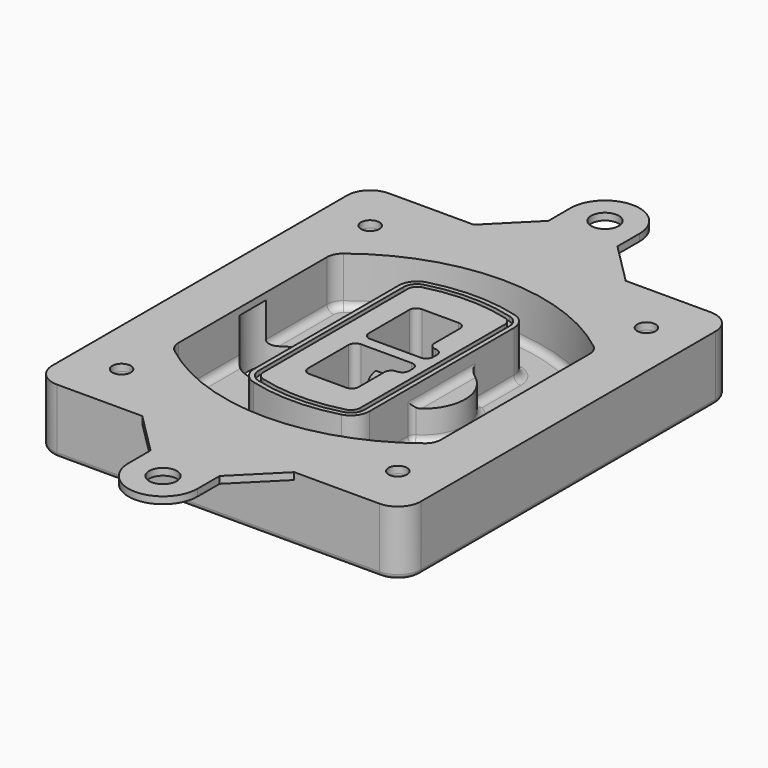
from build123d import *

# Parameters (mm, degrees)
F0_R      = 4
F1_DEPTH  = 25
F2_DEPTH  = 3
F3_DEPTH  = 18
F5_DEPTH  = 21
F6_DEPTH  = 2
F8_DEPTH  = 20
F9_DEPTH  = 16
F10_DEPTH = 25
F7_R      = 6
F7_R_2    = 4
F11_DEPTH = 6
F13_DEPTH = 9
F14_R     = 3
F15_R     = 2
F16_R     = 6
F16_R_2   = 4
F17_DEPTH = 3


with BuildPart() as f1:
    # F0 (on Top) → F1 (new body)
    with BuildSketch(Plane.XY):
        with BuildLine():
            ThreePointArc((-80, -80), (-77.0710678119, -87.0710678119), (-70, -90))
            Line((-70, -90), (70, -90))
            ThreePointArc((70, -90), (77.0710678119, -87.0710678119), (80, -80))
            Line((80, -80), (80, 80))
            ThreePointArc((80, 80), (77.0710678119, 87.0710678119), (70, 90))
            Line((70, 90), (-70, 90))
            ThreePointArc((-70, 90), (-77.0710678119, 87.0710678119), (-80, 80))
            Line((-80, 80), (-80, -80))
        make_face()
        with Locations((-60, -67.5)):
            Circle(F0_R, mode=Mode.SUBTRACT)
        with Locations((60, -67.5)):
            Circle(F0_R, mode=Mode.SUBTRACT)
        with Locations((-60, 67.5)):
            Circle(F0_R, mode=Mode.SUBTRACT)
        with BuildLine():
            ThreePointArc((-64, 40.2934422872), (-62.5820384798, 46.4328484224), (-58.6153846154, 51.3286200352))
            ThreePointArc((-58.6153846154, 51.3286200352), (0, 71.5), (58.6153846154, 51.3286200352))
            ThreePointArc((58.6153846154, 51.3286200352), (62.5820384798, 46.4328484224), (64, 40.2934422872))
            Line((64, 40.2934422872), (64, -40.2934422872))
            ThreePointArc((64, -40.2934422872), (62.5820384798, -46.4328484224), (58.6153846154, -51.3286200352))
            ThreePointArc((58.6153846154, -51.3286200352), (0, -71.5), (-58.6153846154, -51.3286200352))
            ThreePointArc((-58.6153846154, -51.3286200352), (-62.5820384798, -46.4328484224), (-64, -40.2934422872))
            Line((-64, -40.2934422872), (-64, 40.2934422872))
        make_face(mode=Mode.SUBTRACT)
        with Locations((60, 67.5)):
            Circle(F0_R, mode=Mode.SUBTRACT)
        with BuildLine():
            ThreePointArc((58.6153846154, 51.3286200352), (0, 71.5), (-58.6153846154, 51.3286200352))
            ThreePointArc((-58.6153846154, 51.3286200352), (-62.5820384798, 46.4328484224), (-64, 40.2934422872))
            Line((-64, 40.2934422872), (-64, -40.2934422872))
            ThreePointArc((-64, -40.2934422872), (-62.5820384798, -46.4328484224), (-58.6153846154, -51.3286200352))
            ThreePointArc((-58.6153846154, -51.3286200352), (0, -71.5), (58.6153846154, -51.3286200352))
            ThreePointArc((58.6153846154, -51.3286200352), (62.5820384798, -46.4328484224), (64, -40.2934422872))
            Line((64, -40.2934422872), (64, 40.2934422872))
            ThreePointArc((64, 40.2934422872), (62.5820384798, 46.4328484224), (58.6153846154, 51.3286200352))
        make_face()
        with BuildLine():
            Line((-60, -40.2934422872), (-60, 40.2934422872))
            ThreePointArc((-60, 40.2934422872), (-58.9871703427, 44.6787323838), (-56.1538461538, 48.1757121072))
            ThreePointArc((-56.1538461538, 48.1757121072), (0, 67.5), (56.1538461538, 48.1757121072))
            ThreePointArc((56.1538461538, 48.1757121072), (58.9871703427, 44.6787323838), (60, 40.2934422872))
            Line((60, 40.2934422872), (60, -40.2934422872))
            ThreePointArc((60, -40.2934422872), (58.9871703427, -44.6787323838), (56.1538461538, -48.1757121072))
            ThreePointArc((56.1538461538, -48.1757121072), (0, -67.5), (-56.1538461538, -48.1757121072))
            ThreePointArc((-56.1538461538, -48.1757121072), (-58.9871703427, -44.6787323838), (-60, -40.2934422872))
        make_face(mode=Mode.SUBTRACT)
        with BuildLine():
            ThreePointArc((-56.1538461538, 48.1757121072), (-58.9871703427, 44.6787323838), (-60, 40.2934422872))
            Line((-60, 40.2934422872), (-60, -40.2934422872))
            ThreePointArc((-60, -40.2934422872), (-58.9871703427, -44.6787323838), (-56.1538461538, -48.1757121072))
            ThreePointArc((-56.1538461538, -48.1757121072), (0, -67.5), (56.1538461538, -48.1757121072))
            ThreePointArc((56.1538461538, -48.1757121072), (58.9871703427, -44.6787323838), (60, -40.2934422872))
            Line((60, -40.2934422872), (60, 40.2934422872))
            ThreePointArc((60, 40.2934422872), (58.9871703427, 44.6787323838), (56.1538461538, 48.1757121072))
            ThreePointArc((56.1538461538, 48.1757121072), (0, 67.5), (-56.1538461538, 48.1757121072))
        make_face()
        with BuildLine():
            ThreePointArc((54.3076923077, 45.8110311612), (56.2910192399, 43.3631453548), (57, 40.2934422872))
            Line((57, 40.2934422872), (57, -40.2934422872))
            ThreePointArc((57, -40.2934422872), (56.2910192399, -43.3631453548), (54.3076923077, -45.8110311612))
            ThreePointArc((54.3076923077, -45.8110311612), (0, -64.5), (-54.3076923077, -45.8110311612))
            ThreePointArc((-54.3076923077, -45.8110311612), (-56.2910192399, -43.3631453548), (-57, -40.2934422872))
            Line((-57, -40.2934422872), (-57, 40.2934422872))
            ThreePointArc((-57, 40.2934422872), (-56.2910192399, 43.3631453548), (-54.3076923077, 45.8110311612))
            ThreePointArc((-54.3076923077, 45.8110311612), (0, 64.5), (54.3076923077, 45.8110311612))
        make_face(mode=Mode.SUBTRACT)
        with BuildLine():
            Line((57, -40.2934422872), (57, 40.2934422872))
            ThreePointArc((57, 40.2934422872), (56.2910192399, 43.3631453548), (54.3076923077, 45.8110311612))
            ThreePointArc((54.3076923077, 45.8110311612), (0, 64.5), (-54.3076923077, 45.8110311612))
            ThreePointArc((-54.3076923077, 45.8110311612), (-56.2910192399, 43.3631453548), (-57, 40.2934422872))
            Line((-57, 40.2934422872), (-57, -40.2934422872))
            ThreePointArc((-57, -40.2934422872), (-56.2910192399, -43.3631453548), (-54.3076923077, -45.8110311612))
            ThreePointArc((-54.3076923077, -45.8110311612), (0, -64.5), (54.3076923077, -45.8110311612))
            ThreePointArc((54.3076923077, -45.8110311612), (56.2910192399, -43.3631453548), (57, -40.2934422872))
        make_face()
    extrude(amount=-F1_DEPTH)

    # F0 (on Top) → F2 (join)
    with BuildSketch(Plane.XY):
        with BuildLine():
            ThreePointArc((-56.1538461538, 48.1757121072), (-58.9871703427, 44.6787323838), (-60, 40.2934422872))
            Line((-60, 40.2934422872), (-60, -40.2934422872))
            ThreePointArc((-60, -40.2934422872), (-58.9871703427, -44.6787323838), (-56.1538461538, -48.1757121072))
            ThreePointArc((-56.1538461538, -48.1757121072), (0, -67.5), (56.1538461538, -48.1757121072))
            ThreePointArc((56.1538461538, -48.1757121072), (58.9871703427, -44.6787323838), (60, -40.2934422872))
            Line((60, -40.2934422872), (60, 40.2934422872))
            ThreePointArc((60, 40.2934422872), (58.9871703427, 44.6787323838), (56.1538461538, 48.1757121072))
            ThreePointArc((56.1538461538, 48.1757121072), (0, 67.5), (-56.1538461538, 48.1757121072))
        make_face()
        with BuildLine():
            ThreePointArc((54.3076923077, 45.8110311612), (56.2910192399, 43.3631453548), (57, 40.2934422872))
            Line((57, 40.2934422872), (57, -40.2934422872))
            ThreePointArc((57, -40.2934422872), (56.2910192399, -43.3631453548), (54.3076923077, -45.8110311612))
            ThreePointArc((54.3076923077, -45.8110311612), (0, -64.5), (-54.3076923077, -45.8110311612))
            ThreePointArc((-54.3076923077, -45.8110311612), (-56.2910192399, -43.3631453548), (-57, -40.2934422872))
            Line((-57, -40.2934422872), (-57, 40.2934422872))
            ThreePointArc((-57, 40.2934422872), (-56.2910192399, 43.3631453548), (-54.3076923077, 45.8110311612))
            ThreePointArc((-54.3076923077, 45.8110311612), (0, 64.5), (54.3076923077, 45.8110311612))
        make_face(mode=Mode.SUBTRACT)
    extrude(amount=F2_DEPTH)

    # F0 (on Top) → F3 (cut)
    with BuildSketch(Plane.XY):
        with BuildLine():
            Line((57, -40.2934422872), (57, 40.2934422872))
            ThreePointArc((57, 40.2934422872), (56.2910192399, 43.3631453548), (54.3076923077, 45.8110311612))
            ThreePointArc((54.3076923077, 45.8110311612), (0, 64.5), (-54.3076923077, 45.8110311612))
            ThreePointArc((-54.3076923077, 45.8110311612), (-56.2910192399, 43.3631453548), (-57, 40.2934422872))
            Line((-57, 40.2934422872), (-57, -40.2934422872))
            ThreePointArc((-57, -40.2934422872), (-56.2910192399, -43.3631453548), (-54.3076923077, -45.8110311612))
            ThreePointArc((-54.3076923077, -45.8110311612), (0, -64.5), (54.3076923077, -45.8110311612))
            ThreePointArc((54.3076923077, -45.8110311612), (56.2910192399, -43.3631453548), (57, -40.2934422872))
        make_face()
    extrude(amount=-F3_DEPTH, mode=Mode.SUBTRACT)

    # F4 (on face) → F5 (join, through all)
    with BuildSketch(Plane.XY.offset(3)):
        with BuildLine():
            ThreePointArc((-25, -39.2465276821), (-23.3511545998, -44.1109737193), (-19.0842911877, -46.9702398883))
            ThreePointArc((-19.0842911877, -46.9702398883), (0, -49.5), (19.0842911877, -46.9702398883))
            ThreePointArc((19.0842911877, -46.9702398883), (23.3511545998, -44.1109737193), (25, -39.2465276821))
            Line((25, -39.2465276821), (25, 39.2465276821))
            ThreePointArc((25, 39.2465276821), (23.3511545998, 44.1109737193), (19.0842911877, 46.9702398883))
            ThreePointArc((19.0842911877, 46.9702398883), (0, 49.5), (-19.0842911877, 46.9702398883))
            ThreePointArc((-19.0842911877, 46.9702398883), (-23.3511545998, 44.1109737193), (-25, 39.2465276821))
            Line((-25, 39.2465276821), (-25, -39.2465276821))
        make_face()
        with BuildLine():
            ThreePointArc((18.5632183908, 45.0393118368), (21.7633659499, 42.89486221), (23, 39.2465276821))
            Line((23, 39.2465276821), (23, -39.2465276821))
            ThreePointArc((23, -39.2465276821), (21.7633659499, -42.89486221), (18.5632183908, -45.0393118368))
            ThreePointArc((18.5632183908, -45.0393118368), (0, -47.5), (-18.5632183908, -45.0393118368))
            ThreePointArc((-18.5632183908, -45.0393118368), (-21.7633659499, -42.89486221), (-23, -39.2465276821))
            Line((-23, -39.2465276821), (-23, 39.2465276821))
            ThreePointArc((-23, 39.2465276821), (-21.7633659499, 42.89486221), (-18.5632183908, 45.0393118368))
            ThreePointArc((-18.5632183908, 45.0393118368), (0, 47.5), (18.5632183908, 45.0393118368))
        make_face(mode=Mode.SUBTRACT)
        with BuildLine():
            Line((23, -39.2465276821), (23, 39.2465276821))
            ThreePointArc((23, 39.2465276821), (21.7633659499, 42.89486221), (18.5632183908, 45.0393118368))
            ThreePointArc((18.5632183908, 45.0393118368), (0, 47.5), (-18.5632183908, 45.0393118368))
            ThreePointArc((-18.5632183908, 45.0393118368), (-21.7633659499, 42.89486221), (-23, 39.2465276821))
            Line((-23, 39.2465276821), (-23, -39.2465276821))
            ThreePointArc((-23, -39.2465276821), (-21.7633659499, -42.89486221), (-18.5632183908, -45.0393118368))
            ThreePointArc((-18.5632183908, -45.0393118368), (0, -47.5), (18.5632183908, -45.0393118368))
            ThreePointArc((18.5632183908, -45.0393118368), (21.7633659499, -42.89486221), (23, -39.2465276821))
        make_face()
        with BuildLine():
            ThreePointArc((18.0421455939, 43.1083837852), (20.1755772999, 41.6787507007), (21, 39.2465276821))
            Line((21, 39.2465276821), (21, -39.2465276821))
            ThreePointArc((21, -39.2465276821), (20.1755772999, -41.6787507007), (18.0421455939, -43.1083837852))
            ThreePointArc((18.0421455939, -43.1083837852), (0, -45.5), (-18.0421455939, -43.1083837852))
            ThreePointArc((-18.0421455939, -43.1083837852), (-20.1755772999, -41.6787507007), (-21, -39.2465276821))
            Line((-21, -39.2465276821), (-21, 39.2465276821))
            ThreePointArc((-21, 39.2465276821), (-20.1755772999, 41.6787507007), (-18.0421455939, 43.1083837852))
            ThreePointArc((-18.0421455939, 43.1083837852), (0, 45.5), (18.0421455939, 43.1083837852))
        make_face(mode=Mode.SUBTRACT)
        with BuildLine():
            Line((21, -39.2465276821), (21, 39.2465276821))
            ThreePointArc((21, 39.2465276821), (20.1755772999, 41.6787507007), (18.0421455939, 43.1083837852))
            ThreePointArc((18.0421455939, 43.1083837852), (0, 45.5), (-18.0421455939, 43.1083837852))
            ThreePointArc((-18.0421455939, 43.1083837852), (-20.1755772999, 41.6787507007), (-21, 39.2465276821))
            Line((-21, 39.2465276821), (-21, -39.2465276821))
            ThreePointArc((-21, -39.2465276821), (-20.1755772999, -41.6787507007), (-18.0421455939, -43.1083837852))
            ThreePointArc((-18.0421455939, -43.1083837852), (0, -45.5), (18.0421455939, -43.1083837852))
            ThreePointArc((18.0421455939, -43.1083837852), (20.1755772999, -41.6787507007), (21, -39.2465276821))
        make_face()
        with BuildLine():
            Line((-8, -2.5), (14, -2.5))
            ThreePointArc((14, -2.5), (16.1213203436, -3.3786796564), (17, -5.5))
            Line((17, -5.5), (17, -7.5))
            ThreePointArc((17, -7.5), (16.1213203436, -9.6213203436), (14, -10.5))
            ThreePointArc((14, -10.5), (11.8786796564, -11.3786796564), (11, -13.5))
            Line((11, -13.5), (11, -27.5))
            ThreePointArc((11, -27.5), (10.1213203436, -29.6213203436), (8, -30.5))
            Line((8, -30.5), (-8, -30.5))
            ThreePointArc((-8, -30.5), (-10.1213203436, -29.6213203436), (-11, -27.5))
            Line((-11, -27.5), (-11, -5.5))
            ThreePointArc((-11, -5.5), (-10.1213203436, -3.3786796564), (-8, -2.5))
        make_face(mode=Mode.SUBTRACT)
        with BuildLine():
            ThreePointArc((-8, 2.5), (-10.1213203436, 3.3786796564), (-11, 5.5))
            Line((-11, 5.5), (-11, 27.5))
            ThreePointArc((-11, 27.5), (-10.1213203436, 29.6213203436), (-8, 30.5))
            Line((-8, 30.5), (8, 30.5))
            ThreePointArc((8, 30.5), (10.1213203436, 29.6213203436), (11, 27.5))
            Line((11, 27.5), (11, 13.5))
            ThreePointArc((11, 13.5), (11.8786796564, 11.3786796564), (14, 10.5))
            ThreePointArc((14, 10.5), (16.1213203436, 9.6213203436), (17, 7.5))
            Line((17, 7.5), (17, 5.5))
            ThreePointArc((17, 5.5), (16.1213203436, 3.3786796564), (14, 2.5))
            Line((14, 2.5), (-8, 2.5))
        make_face(mode=Mode.SUBTRACT)
    extrude(amount=-F5_DEPTH)

    # F4 (on face) → F6 (cut)
    with BuildSketch(Plane.XY.offset(3)):
        with BuildLine():
            Line((23, -39.2465276821), (23, 39.2465276821))
            ThreePointArc((23, 39.2465276821), (21.7633659499, 42.89486221), (18.5632183908, 45.0393118368))
            ThreePointArc((18.5632183908, 45.0393118368), (0, 47.5), (-18.5632183908, 45.0393118368))
            ThreePointArc((-18.5632183908, 45.0393118368), (-21.7633659499, 42.89486221), (-23, 39.2465276821))
            Line((-23, 39.2465276821), (-23, -39.2465276821))
            ThreePointArc((-23, -39.2465276821), (-21.7633659499, -42.89486221), (-18.5632183908, -45.0393118368))
            ThreePointArc((-18.5632183908, -45.0393118368), (0, -47.5), (18.5632183908, -45.0393118368))
            ThreePointArc((18.5632183908, -45.0393118368), (21.7633659499, -42.89486221), (23, -39.2465276821))
        make_face()
        with BuildLine():
            ThreePointArc((18.0421455939, 43.1083837852), (20.1755772999, 41.6787507007), (21, 39.2465276821))
            Line((21, 39.2465276821), (21, -39.2465276821))
            ThreePointArc((21, -39.2465276821), (20.1755772999, -41.6787507007), (18.0421455939, -43.1083837852))
            ThreePointArc((18.0421455939, -43.1083837852), (0, -45.5), (-18.0421455939, -43.1083837852))
            ThreePointArc((-18.0421455939, -43.1083837852), (-20.1755772999, -41.6787507007), (-21, -39.2465276821))
            Line((-21, -39.2465276821), (-21, 39.2465276821))
            ThreePointArc((-21, 39.2465276821), (-20.1755772999, 41.6787507007), (-18.0421455939, 43.1083837852))
            ThreePointArc((-18.0421455939, 43.1083837852), (0, 45.5), (18.0421455939, 43.1083837852))
        make_face(mode=Mode.SUBTRACT)
    extrude(amount=-F6_DEPTH, mode=Mode.SUBTRACT)

    # F7 (on face) → F8 (join)
    with BuildSketch(Plane(origin=(0, 0, -25), x_dir=(1, 0, 0), z_dir=(0, 0, -1))):
        with BuildLine():
            ThreePointArc((3.28842436, 0), (16.7567035675, 13.4682792075), (30.224982775, 0))
            Line((30.224982775, 0), (35.224982775, 0))
            ThreePointArc((35.224982775, 0), (16.7567035675, 18.4682792075), (-1.71157564, 0))
            Line((-1.71157564, 0), (3.28842436, 0))
        make_face()
        with BuildLine():
            Line((3.28842436, 0), (30.224982775, 0))
            ThreePointArc((30.224982775, 0), (16.7567035675, 13.4682792075), (3.28842436, 0))
        make_face()
        with BuildLine():
            ThreePointArc((3.28842436, 0), (16.7567035675, -13.4682792075), (30.224982775, 0))
            Line((30.224982775, 0), (3.28842436, 0))
        make_face()
        with BuildLine():
            Line((35.224982775, 0), (30.224982775, 0))
            ThreePointArc((30.224982775, 0), (16.7567035675, -13.4682792075), (3.28842436, 0))
            Line((3.28842436, 0), (-1.71157564, 0))
            ThreePointArc((-1.71157564, 0), (16.7567035675, -18.4682792075), (35.224982775, 0))
        make_face()
    extrude(amount=-F8_DEPTH)

    # F7 (on face) → F9 (cut)
    with BuildSketch(Plane(origin=(0, 0, -25), x_dir=(1, 0, 0), z_dir=(0, 0, -1))):
        with BuildLine():
            Line((3.28842436, 0), (30.224982775, 0))
            ThreePointArc((30.224982775, 0), (16.7567035675, 13.4682792075), (3.28842436, 0))
        make_face()
        with BuildLine():
            ThreePointArc((3.28842436, 0), (16.7567035675, -13.4682792075), (30.224982775, 0))
            Line((30.224982775, 0), (3.28842436, 0))
        make_face()
    extrude(amount=-F9_DEPTH, mode=Mode.SUBTRACT)

    # F7 (on face) → F10 (cut)
    with BuildSketch(Plane(origin=(0, 0, -25), x_dir=(1, 0, 0), z_dir=(0, 0, -1))):
        with BuildLine():
            Line((-59.0318229325, 0), (-32.0952645175, 0))
            ThreePointArc((-32.0952645175, 0), (-45.563543725, 13.4682792075), (-59.0318229325, 0))
        make_face()
        with BuildLine():
            ThreePointArc((-59.0318229325, 0), (-45.563543725, -13.4682792075), (-32.0952645175, 0))
            Line((-32.0952645175, 0), (-59.0318229325, 0))
        make_face()
    extrude(amount=-F10_DEPTH, mode=Mode.SUBTRACT)

    # F7 (on face) → F11 (cut)
    with BuildSketch(Plane(origin=(0, 0, -25), x_dir=(1, 0, 0), z_dir=(0, 0, -1))):
        with Locations((60, -67.5)):
            Circle(F7_R)
        with Locations((60, -67.5)):
            Circle(F7_R_2, mode=Mode.SUBTRACT)
        with Locations((-60, -67.5)):
            Circle(F7_R)
        with Locations((-60, -67.5)):
            Circle(F7_R_2, mode=Mode.SUBTRACT)
        with Locations((-60, 67.5)):
            Circle(F7_R)
        with Locations((-60, 67.5)):
            Circle(F7_R_2, mode=Mode.SUBTRACT)
        with Locations((60, 67.5)):
            Circle(F7_R)
        with Locations((60, 67.5)):
            Circle(F7_R_2, mode=Mode.SUBTRACT)
    extrude(amount=-F11_DEPTH, mode=Mode.SUBTRACT)

    # F12 (on face) → F13 (cut, through all)
    with BuildSketch(Plane(origin=(0, 0, -9), x_dir=(1, 0, 0), z_dir=(0, 0, -1))):
        with BuildLine():
            Line((11, 13.5), (11, 17.5481537753))
            ThreePointArc((11, 17.5481537753), (2.5696536419, 11.8239143813), (-1.5415842455, 2.5))
            Line((-1.5415842455, 2.5), (3.5224848595, 2.5))
            ThreePointArc((3.5224848595, 2.5), (6.1857188154, 8.3455872281), (11.2536447004, 12.2927168648))
            ThreePointArc((11.2536447004, 12.2927168648), (11.0640958889, 12.8831798879), (11, 13.5))
        make_face()
        with BuildLine():
            ThreePointArc((11.2536447004, -12.2927168648), (6.1857188154, -8.3455872281), (3.5224848595, -2.5))
            Line((3.5224848595, -2.5), (-1.5415842455, -2.5))
            ThreePointArc((-1.5415842455, -2.5), (2.5696536419, -11.8239143813), (11, -17.5481537753))
            Line((11, -17.5481537753), (11, -13.5))
            ThreePointArc((11, -13.5), (11.0640958889, -12.8831798879), (11.2536447004, -12.2927168648))
        make_face()
        with BuildLine():
            ThreePointArc((11.2536447004, 12.2927168648), (6.1857188154, 8.3455872281), (3.5224848595, 2.5))
            Line((3.5224848595, 2.5), (14, 2.5))
            ThreePointArc((14, 2.5), (16.1213203436, 3.3786796564), (17, 5.5))
            Line((17, 5.5), (17, 7.5))
            ThreePointArc((17, 7.5), (16.1213203436, 9.6213203436), (14, 10.5))
            ThreePointArc((14, 10.5), (12.3601599782, 10.9878446101), (11.2536447004, 12.2927168648))
        make_face()
        with BuildLine():
            Line((14, -2.5), (3.5224848595, -2.5))
            ThreePointArc((3.5224848595, -2.5), (6.1857188154, -8.3455872281), (11.2536447004, -12.2927168648))
            ThreePointArc((11.2536447004, -12.2927168648), (12.3601599782, -10.9878446101), (14, -10.5))
            ThreePointArc((14, -10.5), (16.1213203436, -9.6213203436), (17, -7.5))
            Line((17, -7.5), (17, -5.5))
            ThreePointArc((17, -5.5), (16.1213203436, -3.3786796564), (14, -2.5))
        make_face()
    extrude(amount=F13_DEPTH, mode=Mode.SUBTRACT)

    # F14
    f14_edges = [f1.edges().sort_by_distance(p)[0] for p in [
        (-57, -23.703476, -18),
        (-57, 23.703476, -18),
        (25, 0, -5),
        (25, 16.526506, -11.5),
        (25, -16.526506, -11.5),
        (25, -27.886517, -18),
        (35.224983, 0, -18),
    ]]
    fillet(f14_edges, radius=F14_R)

    # F15
    f15_edges = [f1.edges().sort_by_distance(p)[0] for p in [
        (0, -90, -25),
    ]]
    fillet(f15_edges, radius=F15_R)

    # F16 (on face) → F17 (join)
    with BuildSketch(Plane.XY):
        with BuildLine():
            Line((15, 108), (15, 120))
            ThreePointArc((15, 120), (0, 135), (-15, 120))
            Line((-15, 120), (-15, 108))
            Line((-15, 108), (-33, 90))
            Line((-33, 90), (33, 90))
            Line((33, 90), (15, 108))
        make_face()
        with Locations((0, 120)):
            Circle(F16_R, mode=Mode.SUBTRACT)
        with BuildLine():
            Line((15, -108), (33, -90))
            Line((33, -90), (-33, -90))
            Line((-33, -90), (-15, -108))
            Line((-15, -108), (-15, -120))
            ThreePointArc((-15, -120), (0, -135), (15, -120))
            Line((15, -120), (15, -108))
        make_face()
        with Locations((0, -120)):
            Circle(F16_R, mode=Mode.SUBTRACT)
        with BuildLine():
            Line((70, 90), (33, 90))
            Line((33, 90), (-33, 90))
            Line((-33, 90), (-70, 90))
            ThreePointArc((-70, 90), (-77.0710678119, 87.0710678119), (-80, 80))
            Line((-80, 80), (-80, -80))
            ThreePointArc((-80, -80), (-77.0710678119, -87.0710678119), (-70, -90))
            Line((-70, -90), (-33, -90))
            Line((-33, -90), (33, -90))
            Line((33, -90), (70, -90))
            ThreePointArc((70, -90), (77.0710678119, -87.0710678119), (80, -80))
            Line((80, -80), (80, 80))
            ThreePointArc((80, 80), (77.0710678119, 87.0710678119), (70, 90))
        make_face()
        with Locations((-60, -67.5)):
            Circle(F16_R_2, mode=Mode.SUBTRACT)
        with Locations((60, -67.5)):
            Circle(F16_R_2, mode=Mode.SUBTRACT)
        with Locations((-60, 67.5)):
            Circle(F16_R_2, mode=Mode.SUBTRACT)
        with BuildLine():
            ThreePointArc((-60, 40.2934422872), (-58.9871703427, 44.6787323838), (-56.1538461538, 48.1757121072))
            ThreePointArc((-56.1538461538, 48.1757121072), (0, 67.5), (56.1538461538, 48.1757121072))
            ThreePointArc((56.1538461538, 48.1757121072), (58.9871703427, 44.6787323838), (60, 40.2934422872))
            Line((60, 40.2934422872), (60, -40.2934422872))
            ThreePointArc((60, -40.2934422872), (58.9871703427, -44.6787323838), (56.1538461538, -48.1757121072))
            ThreePointArc((56.1538461538, -48.1757121072), (0, -67.5), (-56.1538461538, -48.1757121072))
            ThreePointArc((-56.1538461538, -48.1757121072), (-58.9871703427, -44.6787323838), (-60, -40.2934422872))
            Line((-60, -40.2934422872), (-60, 40.2934422872))
        make_face(mode=Mode.SUBTRACT)
        with Locations((60, 67.5)):
            Circle(F16_R_2, mode=Mode.SUBTRACT)
    extrude(amount=F17_DEPTH)


solid = f1.part
